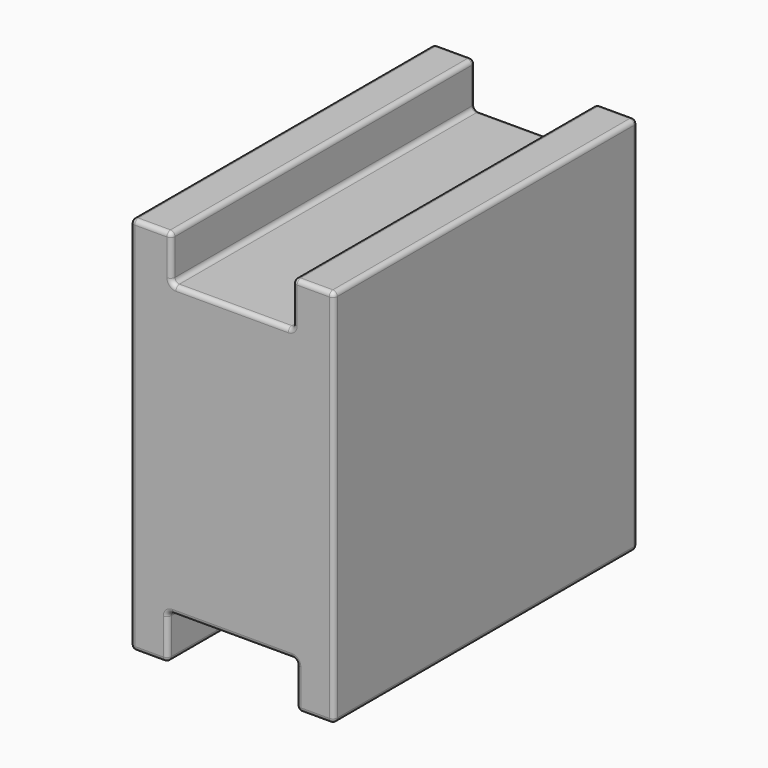
from build123d import *

# Parameters (mm, degrees)
F1_DEPTH = 12.7
F2_R     = 0.3


# Not quite as in the source:
# - a feature names something its author has since deleted; it is built from what else it names


with BuildPart() as f1:
    # F0 (on Front) → F1 (new body, symmetric)
    with BuildSketch(Plane.XZ):
        Polygon((0, 25.4), (0, 0), (2.5, 0), (2.5, 3), (11.1, 3), (11.1, 0), (13.6, 0), (13.6, 25.4), (10.855, 25.4), (10.855, 22.4), (2.745, 22.4), (2.745, 25.4), align=None)
    extrude(amount=F1_DEPTH, both=True)

    # F2
    f2_edges = [f1.edges().sort_by_distance(p)[0] for p in [
        (0, 12.7, 12.7),
        (0, -12.7, 12.7),
        (0, 0, 0),
        (1.25, -12.7, 0),
        (13.6, -12.7, 12.7),
        (13.6, 12.7, 12.7),
        (1.25, 12.7, 0),
        (6.8, -12.7, 22.4),
        (2.745, -12.7, 23.9),
        (2.745, 0, 25.4),
        (10.855, -12.7, 23.9),
        (10.855, 0, 25.4),
        (2.745, 0, 22.4),
        (6.8, 12.7, 22.4),
        (10.855, 0, 22.4),
        (2.5, 0, 3),
        (2.5, -12.7, 1.5),
        (6.8, -12.7, 3),
        (11.1, -12.7, 1.5),
        (11.1, 0, 0),
        (12.35, -12.7, 0),
        (2.5, 12.7, 1.5),
        (6.8, 12.7, 3),
        (11.1, 12.7, 1.5),
        (11.1, 0, 3),
        (12.2275, -12.7, 25.4),
        (1.3725, -12.7, 25.4),
        (1.3725, 12.7, 25.4),
        (12.2275, 12.7, 25.4),
        (12.35, 12.7, 0),
        (0, 0, 25.4),
        (2.745, 12.7, 23.9),
        (10.855, 12.7, 23.9),
        (13.6, 0, 25.4),
        (13.6, 0, 0),
        (2.5, 0, 0),
    ]]
    fillet(f2_edges, radius=F2_R)


solid = f1.part
